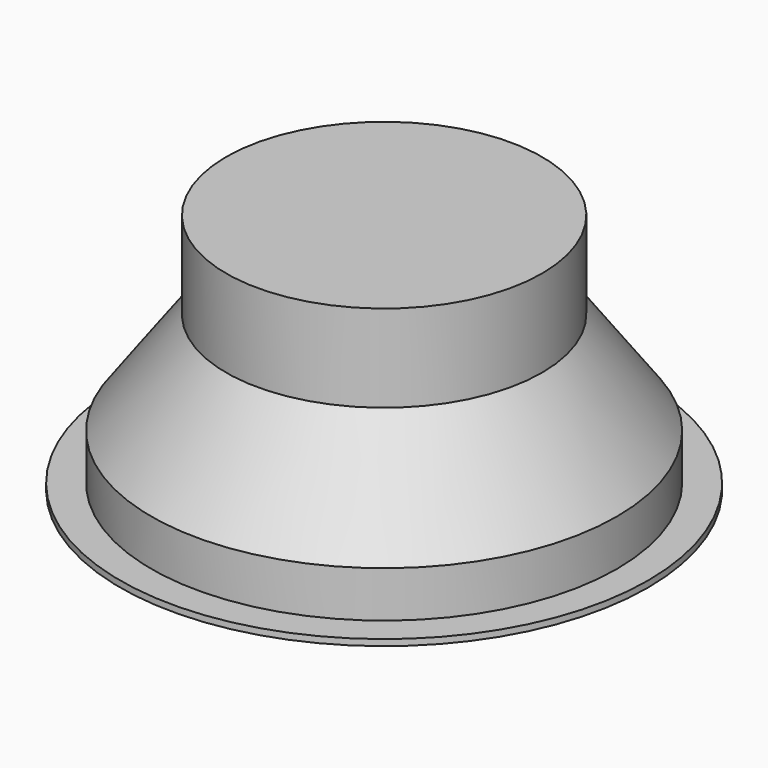
from build123d import *

# Parameters (mm, degrees)
F0_R     = 93.3
F0_R_2   = 90.8
F1_DEPTH = 21
F0_R_3   = 105.8
F2_DEPTH = 2.5
F3_R     = 90.8
F4_DEPTH = 2.5
F3_R_2   = 93.3
F5_DEPTH = 41
F6_SIZE2 = 40.99999
F6_SIZE  = 29.99999
F7_DEPTH = 35


# Not quite as in the source:
# - a fillet or chamfer is up to 0.001 mm smaller than in the source, because OpenCascade refuses the exact size


with BuildPart() as f1:
    # F0 (on Top) → F1 (new body)
    with BuildSketch(Plane.XY):
        Circle(F0_R)
        Circle(F0_R_2, mode=Mode.SUBTRACT)
    extrude(amount=F1_DEPTH)

    # F0 (on Top) → F2 (join)
    with BuildSketch(Plane.XY):
        Circle(F0_R_3)
        Circle(F0_R, mode=Mode.SUBTRACT)
    extrude(amount=F2_DEPTH)


with BuildPart() as f4:
    # F3 (on face) → F4 (new body)
    with BuildSketch(Plane.XY.offset(21)):
        Circle(F3_R)
    extrude(amount=-F4_DEPTH)


with BuildPart() as f5:
    # F3 (on face) → F5 (new body)
    with BuildSketch(Plane.XY.offset(21)):
        Circle(F3_R_2)
        Circle(F3_R, mode=Mode.SUBTRACT)
        Circle(F3_R)
    extrude(amount=F5_DEPTH)

    # F6 (size 30 and 41 in the source; OpenCascade refuses exactly that, so slightly less here)
    f6_edges = [f5.edges().sort_by_distance(p)[0] for p in [
        (-93.3, 0, 62),
    ]]
    f6_side = f5.faces().sort_by_distance((0, 0, 62))[0]
    chamfer(f6_edges, length=F6_SIZE, length2=F6_SIZE2, reference=f6_side)

    # F7 (add): a face of the model
    f7_faces = [f5.faces().sort_by_distance(p)[0] for p in [
        (0, 0, 62),
    ]]
    extrude(f7_faces, amount=F7_DEPTH)


solid = Compound([f1.part, f4.part, f5.part])
